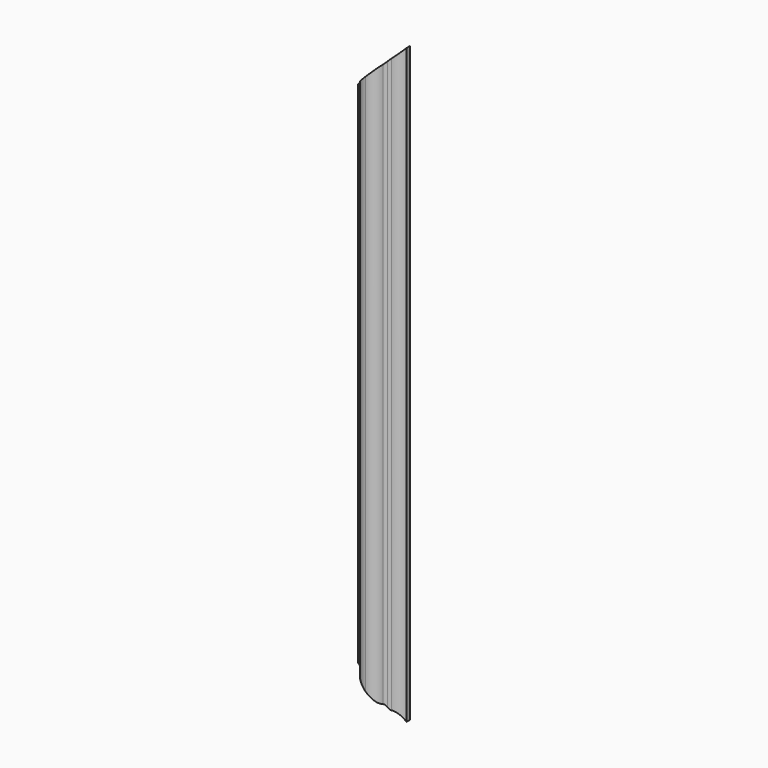
from build123d import *

# Parameters (mm, degrees)
F1_DEPTH = 225.425
F2_R     = 2.54
F3_R     = 2.54
F4_R     = 2.54
F6_DEPTH = 17.4635001
F8_DEPTH = 6.35


# Not quite as in the source:
# - ends of sketch curves that miss each other by under 0.0002 mm in the source are joined


with BuildPart() as f1:
    # F0 (on Top) → F1 (new body, symmetric)
    with BuildSketch(Plane.XY):
        with BuildLine():
            Line((15.875, 5.55625), (15.875, 8.73125))
            Line((15.875, 8.73125), (-15.875, 8.73125))
            Line((-15.875, 8.73125), (-15.875, -0.79375))
            Line((-15.875, -0.79375), (-12.7, -0.79375))
            ThreePointArc((-12.7, -0.79375), (-9.8710707302, -6.4481459867), (-3.9751, -8.73125))
            Line((-3.9751, -8.73125), (-3.96875, -8.73125))
            ThreePointArc((-3.96875, -8.73125), (1.9312218072, -6.4502821485), (4.7625, -0.79375))
            Line((4.7625, -0.79375), (7.9375, -0.79375))
            ThreePointArc((7.9375, -0.79375), (10.9883747468, 3.5285940665), (15.875, 5.55625))
        make_face()
    extrude(amount=F1_DEPTH, both=True)

    # F2
    f2_edges = [f1.edges().sort_by_distance(p)[0] for p in [
        (7.9375, -0.79375, 0),
    ]]
    fillet(f2_edges, radius=F2_R)

    # F3
    f3_edges = [f1.edges().sort_by_distance(p)[0] for p in [
        (-12.7, -0.79375, 0),
    ]]
    fillet(f3_edges, radius=F3_R)

    # F4
    f4_edges = [f1.edges().sort_by_distance(p)[0] for p in [
        (4.7625, -0.79375, 0),
    ]]
    fillet(f4_edges, radius=F4_R)

    # F5 (on face) → F6 (cut, through all)
    with BuildSketch(Plane(origin=(0, 8.73125, 0), x_dir=(-1, 0, 0), z_dir=(0, 1, 0))):
        Polygon((15.875, 225.425), (-15.875, 225.425), (15.875, 193.675), align=None)
        Polygon((15.875, -193.675), (-15.875, -225.425), (15.875, -225.425), align=None)
    extrude(amount=-F6_DEPTH, mode=Mode.SUBTRACT)

    # F7 (on face) → F8 (cut)
    with BuildSketch(Plane(origin=(0, 8.73125, 0), x_dir=(-1, 0, 0), z_dir=(0, 1, 0))):
        Polygon((15.875, 193.675), (9.525, 200.025), (9.525, -200.025), (15.875, -193.675), align=None)
    extrude(amount=-F8_DEPTH, mode=Mode.SUBTRACT)


solid = f1.part
